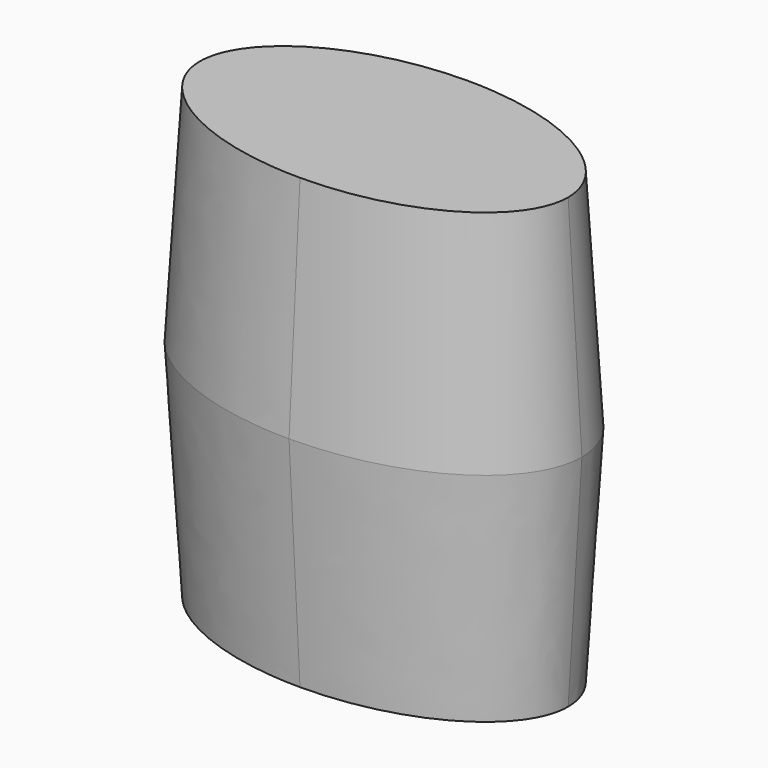
from build123d import *

# Parameters (mm, degrees)
F1_DEPTH      = 85
F1_TAPER      = 3.5
F1_DEPTH_BACK = 85
F1_TAPER_BACK = 3.5


with BuildPart() as f1:
    # F0 (on Top) → F1 (new body, two sides)
    with BuildSketch(Plane.XY) as f1_sk:
        with BuildLine():
            add(Edge.make_bspline(
                [(0, 45), (-129.9038105677, 45), (-64.9519052838, -22.5), (0, -90), (64.9519052838, -22.5), (129.9038105677, 45), (0, 45)],
                knots=[4.7123889804, 4.7123889804, 4.7123889804, 6.8067840828, 6.8067840828, 8.9011791852, 8.9011791852, 10.9955742876, 10.9955742876, 10.9955742876], degree=2, weights=[1, 0.5, 1, 0.5, 1, 0.5, 1]))
        make_face()
    extrude(amount=F1_DEPTH, taper=F1_TAPER)
    extrude(f1_sk.sketch, amount=-F1_DEPTH_BACK, taper=F1_TAPER_BACK)


solid = f1.part
